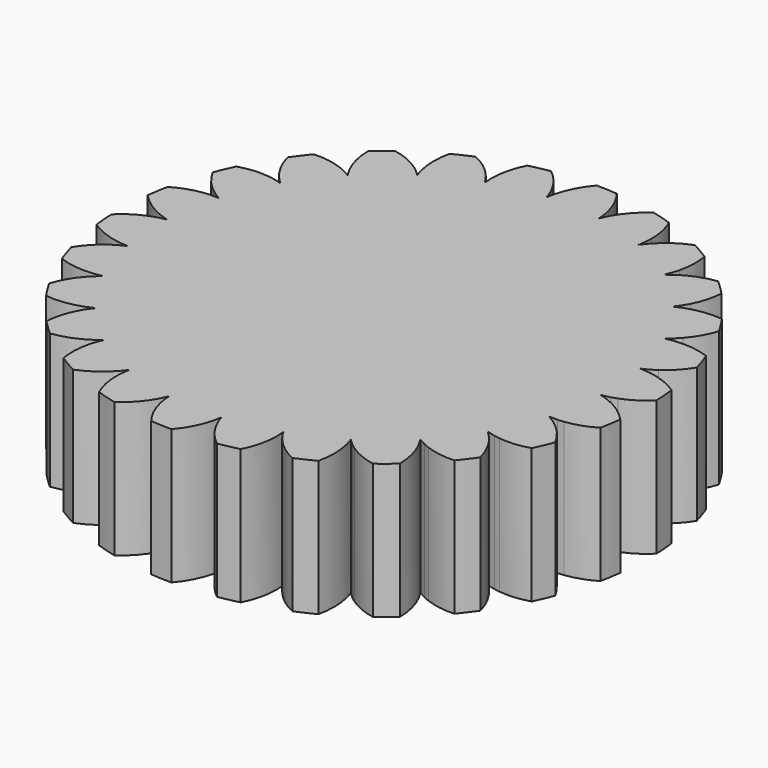
from build123d import *

# Parameters (mm, degrees)
F1_DEPTH = 12.7
F2_COUNT = 26


with BuildPart() as f1:
    # F0 (on Top) → F1 (new body)
    with BuildSketch(Plane.XY):
        with BuildLine():
            ThreePointArc((7.9296197565, 23.5951858335), (6.9911317973, 23.8900761864), (6.0417249702, 24.1476546146))
            ThreePointArc((6.0417249702, 24.1476546146), (4.3226425573, 22.4330749308), (3.2648662162, 20.2476374354))
            ThreePointArc((3.2648662162, 20.2476374354), (5.7837443287, 19.6767495961), (8.2108987358, 18.7938105523))
            ThreePointArc((8.2108987358, 18.7938105523), (8.3954934616, 19.5156536929), (8.4994507341, 20.2534379554))
            ThreePointArc((8.4994507341, 20.2534379554), (8.5176465567, 20.5391701676), (8.5237154667, 20.8254168329))
            ThreePointArc((8.5237154667, 20.8254168329), (8.373521449, 22.2418004346), (7.9296197565, 23.5951858335))
        make_face()
        with BuildLine():
            ThreePointArc((4.0264902572, 14.4598933509), (-1.7431476836, 15.057566034), (-4.9211585336, 19.9100068261))
            ThreePointArc((-4.9211585336, 19.9100068261), (-12.6431262329, -16.1486077476), (20.5091729021, 0))
            ThreePointArc((20.5091729021, 0), (19.2415803806, 7.0984334598), (15.5954927821, 13.3194135761))
            ThreePointArc((15.5954927821, 13.3194135761), (9.5256046991, 10.9946956396), (4.0264902572, 14.4598933509))
        make_face()
        with BuildLine():
            ThreePointArc((3.2648662162, 20.2476374354), (-0.8451772993, 20.4917507417), (-4.9211585336, 19.9100068261))
            ThreePointArc((-4.9211585336, 19.9100068261), (-1.7431476836, 15.057566034), (4.0264902572, 14.4598933509))
            ThreePointArc((4.0264902572, 14.4598933509), (3.0384725246, 17.2738616412), (3.2648662162, 20.2476374354))
        make_face()
        with BuildLine():
            ThreePointArc((4.0264902572, 14.4598933509), (9.5256046991, 10.9946956396), (15.5954927821, 13.3194135761))
            ThreePointArc((15.5954927821, 13.3194135761), (12.2138579016, 16.4756744411), (8.2108987358, 18.7938105523))
            ThreePointArc((8.2108987358, 18.7938105523), (6.6287005247, 16.1344397874), (4.0264902572, 14.4598933509))
        make_face()
        with BuildLine():
            ThreePointArc((8.2108987358, 18.7938105523), (5.7837443287, 19.6767495961), (3.2648662162, 20.2476374354))
            ThreePointArc((3.2648662162, 20.2476374354), (3.0384725246, 17.2738616412), (4.0264902572, 14.4598933509))
            ThreePointArc((4.0264902572, 14.4598933509), (6.6287005247, 16.1344397874), (8.2108987358, 18.7938105523))
        make_face()
    extrude(amount=F1_DEPTH)

    # F2: F1 ×26 about axis
    f2_axis = Axis((0, 0, 12.7), (0, 0, 1))


with BuildPart() as f1_1:
    add(f1.part)
    for i in range(1, F2_COUNT):
        add(f1.part.rotate(f2_axis, i * 360 / F2_COUNT))


solid = f1_1.part
